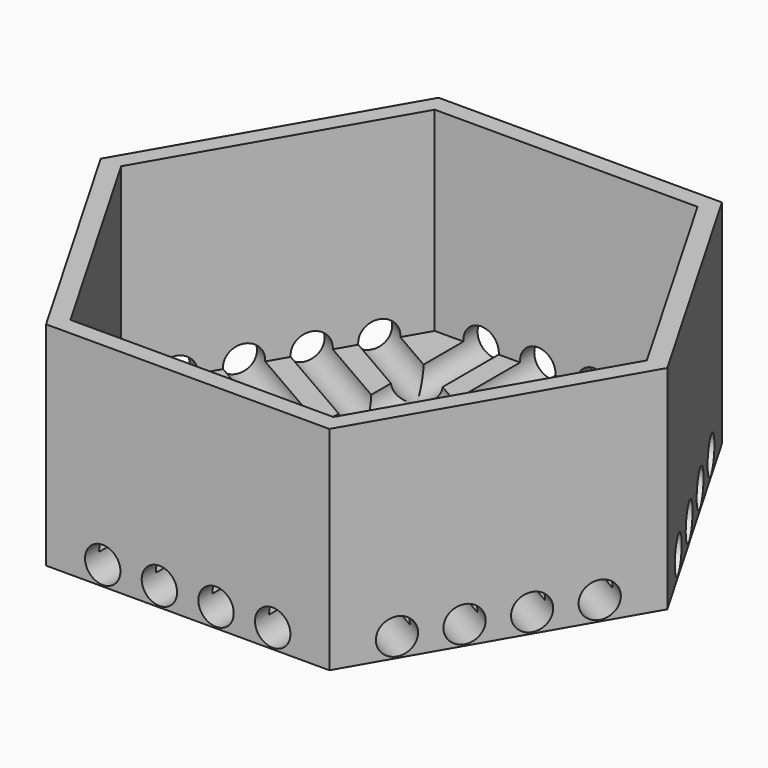
from build123d import *

# Parameters (mm, degrees)
F2_DEPTH = 76.2
F3_T     = -6.35
F4_R     = 6.35
F5_DEPTH = 203.2
F6_R     = 6.35
F7_DEPTH = 203.2
F8_R     = 6.35
F9_DEPTH = 203.2


with BuildPart() as f2:
    # F0 (on Top) → F2 (new body)
    with BuildSketch(Plane.XY):
        Polygon((-50.8, 87.9881810245), (-101.6, 0), (-50.8, -87.9881810245), (50.8, -87.9881810245), (101.6, 0), (50.8, 87.9881810245), align=None)
    extrude(amount=F2_DEPTH)

    # F3
    f3_openings = [f2.faces().sort_by_distance(p)[0] for p in [
        (0, 0, 76.2),
    ]]
    offset(amount=F3_T, openings=f3_openings)

    # F4 (on face) → F5 (cut)
    with BuildSketch(Plane(origin=(76.2, 43.9940905122, 0), x_dir=(-0.5, 0.8660254038, 0), z_dir=(0.8660254038, 0.5, 0))):
        with Locations((-30.48, 6.858)):
            Circle(F4_R)
        with Locations((-10.16, 6.858)):
            Circle(F4_R)
        with Locations((10.16, 6.858)):
            Circle(F4_R)
        with Locations((30.48, 6.858)):
            Circle(F4_R)
    extrude(amount=-F5_DEPTH, mode=Mode.SUBTRACT)

    # F6 (on face) → F7 (cut)
    with BuildSketch(Plane(origin=(-76.2, 43.9940905122, 0), x_dir=(-0.5, -0.8660254038, 0), z_dir=(-0.8660254038, 0.5, 0))):
        with Locations((-30.48, 6.858)):
            Circle(F6_R)
        with Locations((-10.16, 6.858)):
            Circle(F6_R)
        with Locations((10.16, 6.858)):
            Circle(F6_R)
        with Locations((30.48, 6.858)):
            Circle(F6_R)
    extrude(amount=-F7_DEPTH, mode=Mode.SUBTRACT)

    # F8 (on face) → F9 (cut)
    with BuildSketch(Plane(origin=(0, 87.9881810245, 0), x_dir=(-1, 0, 0), z_dir=(0, 1, 0))):
        with Locations((-30.48, 6.858)):
            Circle(F8_R)
        with Locations((-10.16, 6.858)):
            Circle(F8_R)
        with Locations((10.16, 6.858)):
            Circle(F8_R)
        with Locations((30.48, 6.858)):
            Circle(F8_R)
    extrude(amount=-F9_DEPTH, mode=Mode.SUBTRACT)


solid = f2.part
